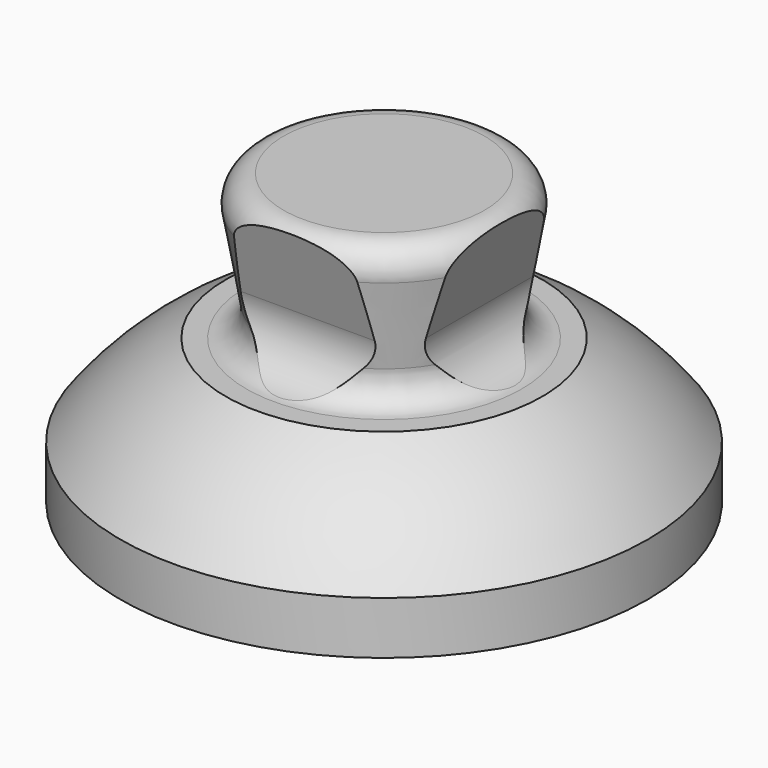
from build123d import *

# Parameters (mm, degrees)
F0_R            = 20
F1_DEPTH        = 4
F4_R            = 2
F5_R            = 2
F7_DEPTH        = 20.001
F7_DEPTH_BACK   = 20.001
F7_COPIES_COUNT = 4


# Not quite as in the source:
# - a pattern or mirror of a feature is missing from the dataset's text; its kind, count and spacing are read off the source's solid


with BuildPart() as f1:
    # F0 (on Top) → F1 (new body)
    with BuildSketch(Plane.XY):
        Circle(F0_R)
    extrude(amount=F1_DEPTH)

    # F2 (on Right) → F3 (revolve)
    with BuildSketch(Plane.YZ):
        with BuildLine():
            Line((0, 10.9317121995), (0, 4))
            Line((0, 4), (20, 4))
            ThreePointArc((20, 4), (16.371076889, 7.8941218768), (12, 10.9317121995))
            Line((12, 10.9317121995), (8.0604032122, 10.9317121995))
            Line((8.0604032122, 10.9317121995), (0, 10.9317121995))
        make_face()
        Polygon((0, 21.9317121995), (0, 10.9317121995), (8.0604032122, 10.9317121995), (10, 21.9317121995), align=None)
    revolve(axis=Axis((0, 0, 7.4658560997), (0, 0, -1)))

    # F4
    f4_edges = [f1.edges().sort_by_distance(p)[0] for p in [
        (0, -8.060403, 10.931712),
    ]]
    fillet(f4_edges, radius=F4_R)

    # F5
    f5_edges = [f1.edges().sort_by_distance(p)[0] for p in [
        (0, -10, 21.931712),
    ]]
    fillet(f5_edges, radius=F5_R)

    # F6 (on Right) → F7 (cut, two sides)
    with BuildSketch(Plane.YZ) as f7_sk:
        with BuildLine():
            Line((-12, 21.9317121995), (-12, 10.9317121995))
            Line((-12, 10.9317121995), (-10.6138476882, 10.9317121995))
            ThreePointArc((-10.6138476882, 10.9317121995), (-7.8371109972, 12.3010471979), (-7.2331072962, 15.3375788573))
            Line((-7.2331072962, 15.3375788573), (-9, 21.9317121995))
            Line((-9, 21.9317121995), (-12, 21.9317121995))
        make_face()
    f7 = extrude(amount=F7_DEPTH, mode=Mode.SUBTRACT) + extrude(f7_sk.sketch, amount=-F7_DEPTH_BACK, mode=Mode.SUBTRACT)

    # F7_copies: F7 ×4 about axis
    f7_copies_axis = Axis((0, 0, 0), (0, 0, 1))
    for i in range(1, F7_COPIES_COUNT):
        add(f7.rotate(f7_copies_axis, i * 360 / F7_COPIES_COUNT), mode=Mode.SUBTRACT)


solid = f1.part
